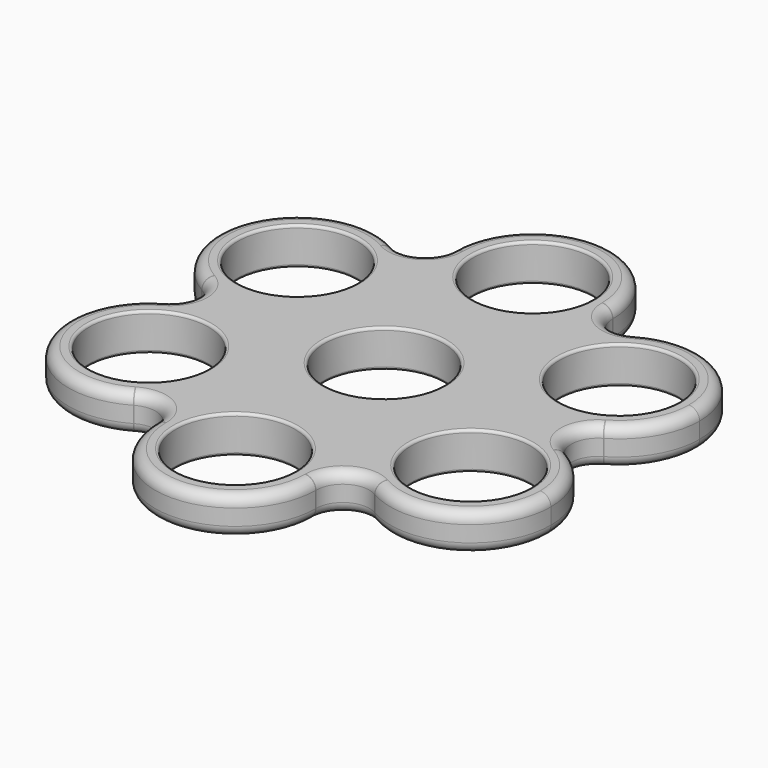
from build123d import *

# Parameters (mm, degrees)
F0_R     = 11.175
F1_DEPTH = 7
F2_R     = 5
F3_R     = 0.5
F4_R     = 2


# Not quite as in the source:
# - a feature names something its author has since deleted; it is built from what else it names


with BuildPart() as f1:
    # F0 (on Top) → F1 (new body)
    with BuildSketch(Plane.XY):
        with BuildLine():
            Line((15, 0), (15, 8.6602540378))
            Line((15, 8.6602540378), (7.5, 12.9903810568))
            Line((7.5, 12.9903810568), (0, 17.3205080757))
            Line((0, 17.3205080757), (-7.5, 12.9903810568))
            Line((-7.5, 12.9903810568), (-15, 8.6602540378))
            Line((-15, 8.6602540378), (-15, 0))
            Line((-15, 0), (-11.175, 0))
            ThreePointArc((-11.175, 0), (0, 11.175), (11.175, 0))
            Line((11.175, 0), (15, 0))
        make_face()
        with BuildLine():
            Line((15, 25.9807621135), (15, 34.7227789462))
            ThreePointArc((15, 34.7227789462), (0, 19.7227789462), (-15, 34.7227789462))
            Line((-15, 34.7227789462), (-15, 25.9807621135))
            Line((-15, 25.9807621135), (0, 17.3205080757))
            Line((0, 17.3205080757), (15, 25.9807621135))
        make_face()
        with BuildLine():
            ThreePointArc((-15, 34.7227789462), (0, 19.7227789462), (15, 34.7227789462))
            ThreePointArc((15, 34.7227789462), (0, 49.7227789462), (-15, 34.7227789462))
        make_face()
        with Locations((0, 34.7227789462)):
            Circle(F0_R, mode=Mode.SUBTRACT)
        with BuildLine():
            ThreePointArc((-15.0708086574, 17.3613894731), (-17.0804276006, 24.8613894731), (-22.5708086574, 30.3517705298))
            ThreePointArc((-22.5708086574, 30.3517705298), (-43.0611897141, 24.8613894731), (-37.5708086574, 4.3710084163))
            ThreePointArc((-37.5708086574, 4.3710084163), (-22.5708086574, 4.3710084163), (-15.0708086574, 17.3613894731))
        make_face()
        with Locations((-30.0708086574, 17.3613894731)):
            Circle(F0_R, mode=Mode.SUBTRACT)
        with BuildLine():
            ThreePointArc((-15, -34.7227789462), (0, -49.7227789462), (15, -34.7227789462))
            ThreePointArc((15, -34.7227789462), (0, -19.7227789462), (-15, -34.7227789462))
        make_face()
        with Locations((0, -34.7227789462)):
            Circle(F0_R, mode=Mode.SUBTRACT)
        with BuildLine():
            Line((15, -34.7227789462), (15, -25.9807621135))
            Line((15, -25.9807621135), (0, -17.3205080757))
            Line((0, -17.3205080757), (-15, -25.9807621135))
            Line((-15, -25.9807621135), (-15, -34.7227789462))
            ThreePointArc((-15, -34.7227789462), (0, -19.7227789462), (15, -34.7227789462))
        make_face()
        Polygon((30, 0), (15, 8.6602540378), (15, 0), (15, -8.6602540378), align=None)
        with BuildLine():
            ThreePointArc((-15.0708086574, -17.3613894731), (-22.5708086574, -4.3710084163), (-37.5708086574, -4.3710084163))
            ThreePointArc((-37.5708086574, -4.3710084163), (-43.0611897141, -24.8613894731), (-22.5708086574, -30.3517705298))
            ThreePointArc((-22.5708086574, -30.3517705298), (-17.0804276006, -24.8613894731), (-15.0708086574, -17.3613894731))
        make_face()
        with Locations((-30.0708086574, -17.3613894731)):
            Circle(F0_R, mode=Mode.SUBTRACT)
        with BuildLine():
            Line((-15, -8.6602540378), (-30, 0))
            Line((-30, 0), (-37.5708086574, -4.3710084163))
            ThreePointArc((-37.5708086574, -4.3710084163), (-22.5708086574, -4.3710084163), (-15.0708086574, -17.3613894731))
            ThreePointArc((-15.0708086574, -17.3613894731), (-17.0804276006, -24.8613894731), (-22.5708086574, -30.3517705298))
            Line((-22.5708086574, -30.3517705298), (-15, -25.9807621135))
            Line((-15, -25.9807621135), (-15, -8.6602540378))
        make_face()
        Polygon((-15, 0), (-15, 8.6602540378), (-30, 0), (-15, -8.6602540378), align=None)
        with BuildLine():
            Line((-15, 8.6602540378), (-15, 25.9807621135))
            Line((-15, 25.9807621135), (-22.5708086574, 30.3517705298))
            ThreePointArc((-22.5708086574, 30.3517705298), (-17.0804276006, 24.8613894731), (-15.0708086574, 17.3613894731))
            ThreePointArc((-15.0708086574, 17.3613894731), (-22.5708086574, 4.3710084163), (-37.5708086574, 4.3710084163))
            Line((-37.5708086574, 4.3710084163), (-30, 0))
            Line((-30, 0), (-15, 8.6602540378))
        make_face()
        Polygon((0, 17.3205080757), (-15, 25.9807621135), (-15, 8.6602540378), (-7.5, 12.9903810568), align=None)
        with BuildLine():
            Line((15, -8.6602540378), (15, 0))
            Line((15, 0), (11.175, 0))
            ThreePointArc((11.175, 0), (0, -11.175), (-11.175, 0))
            Line((-11.175, 0), (-15, 0))
            Line((-15, 0), (-15, -8.6602540378))
            Line((-15, -8.6602540378), (-7.5, -12.9903810568))
            Line((-7.5, -12.9903810568), (0, -17.3205080757))
            Line((0, -17.3205080757), (7.5, -12.9903810568))
            Line((7.5, -12.9903810568), (15, -8.6602540378))
        make_face()
        Polygon((15, 8.6602540378), (15, 25.9807621135), (0, 17.3205080757), (7.5, 12.9903810568), align=None)
        with BuildLine():
            Line((22.5708086574, 30.3517705298), (15, 25.9807621135))
            Line((15, 25.9807621135), (15, 8.6602540378))
            Line((15, 8.6602540378), (30, 0))
            Line((30, 0), (37.5708086574, 4.3710084163))
            ThreePointArc((37.5708086574, 4.3710084163), (17.0804276006, 9.8613894731), (22.5708086574, 30.3517705298))
        make_face()
        with BuildLine():
            ThreePointArc((45.0708086574, 17.3613894731), (37.5708086574, 30.3517705298), (22.5708086574, 30.3517705298))
            ThreePointArc((22.5708086574, 30.3517705298), (17.0804276006, 9.8613894731), (37.5708086574, 4.3710084163))
            ThreePointArc((37.5708086574, 4.3710084163), (43.0611897141, 9.8613894731), (45.0708086574, 17.3613894731))
        make_face()
        with Locations((30.0708086574, 17.3613894731)):
            Circle(F0_R, mode=Mode.SUBTRACT)
        with BuildLine():
            ThreePointArc((45.0708086574, -17.3613894731), (43.0611897141, -9.8613894731), (37.5708086574, -4.3710084163))
            ThreePointArc((37.5708086574, -4.3710084163), (17.0804276006, -9.8613894731), (22.5708086574, -30.3517705298))
            ThreePointArc((22.5708086574, -30.3517705298), (37.5708086574, -30.3517705298), (45.0708086574, -17.3613894731))
        make_face()
        with Locations((30.0708086574, -17.3613894731)):
            Circle(F0_R, mode=Mode.SUBTRACT)
        Polygon((15, -25.9807621135), (15, -8.6602540378), (7.5, -12.9903810568), (0, -17.3205080757), align=None)
        Polygon((-7.5, -12.9903810568), (-15, -8.6602540378), (-15, -25.9807621135), (0, -17.3205080757), align=None)
        with BuildLine():
            Line((37.5708086574, -4.3710084163), (30, 0))
            Line((30, 0), (15, -8.6602540378))
            Line((15, -8.6602540378), (15, -25.9807621135))
            Line((15, -25.9807621135), (22.5708086574, -30.3517705298))
            ThreePointArc((22.5708086574, -30.3517705298), (17.0804276006, -9.8613894731), (37.5708086574, -4.3710084163))
        make_face()
    extrude(amount=F1_DEPTH)

    # F2
    f2_edges = [f1.edges().sort_by_distance(p)[0] for p in [
        (-15, -25.980762, 3.5),
        (-30, 0, 3.5),
        (30, 0, 3.5),
        (15, -25.980762, 3.5),
        (15, 25.980762, 3.5),
        (-15, 25.980762, 3.5),
    ]]
    fillet(f2_edges, radius=F2_R)

    # F3
    f3_edges = [f1.edges().sort_by_distance(p)[0] for p in [
        (-11.175, 34.722779, 7),
        (-11.175, 0, 7),
        (-11.175, 34.722779, 0),
        (-11.175, 0, 0),
        (-41.245809, -17.361389, 7),
        (-41.245809, 17.361389, 0),
        (-11.175, -34.722779, 0),
        (-41.245809, -17.361389, 0),
        (-11.175, -34.722779, 7),
        (-41.245809, 17.361389, 7),
        (18.895809, 17.361389, 7),
        (18.895809, -17.361389, 7),
        (18.895809, 17.361389, 0),
        (18.895809, -17.361389, 0),
    ]]
    fillet(f3_edges, radius=F3_R)

    # F4
    f4_edges = [f1.edges().sort_by_distance(p)[0] for p in [
        (-17.5, 30.310889, 0),
        (-15, 34.641016, 3.5),
        (-22.5, 30.310889, 3.5),
        (-17.5, 30.310889, 7),
        (-15, 34.681898, 0),
        (-15, 34.722779, 3.5),
        (-15, 34.681898, 7),
        (15, 34.722779, 3.5),
        (0, 49.722779, 0),
        (0, 49.722779, 7),
        (15, 34.681898, 0),
        (15, 34.641016, 3.5),
        (15, 34.681898, 7),
        (17.5, 30.310889, 0),
        (22.5, 30.310889, 3.5),
        (17.5, 30.310889, 7),
        (-43.06119, -24.861389, 7),
        (-43.06119, -24.861389, 0),
        (-22.535404, -30.33133, 0),
        (-17.5, -30.310889, 0),
        (-15, -34.681898, 0),
        (-37.535404, -4.350568, 0),
        (0, -49.722779, 0),
        (-35, 0, 0),
        (15, -34.681898, 0),
        (-37.535404, 4.350568, 0),
        (17.5, -30.310889, 0),
        (-43.06119, 24.861389, 0),
        (22.535404, -30.33133, 0),
        (-22.535404, 30.33133, 0),
        (43.06119, -24.861389, 0),
        (37.535404, -4.350568, 0),
        (35, 0, 0),
        (37.535404, 4.350568, 0),
        (43.06119, 24.861389, 0),
        (22.535404, 30.33133, 0),
        (-22.535404, -30.33133, 7),
        (-17.5, -30.310889, 7),
        (-15, -34.681898, 7),
        (-37.535404, -4.350568, 7),
        (0, -49.722779, 7),
        (-35, 0, 7),
        (15, -34.681898, 7),
        (-37.535404, 4.350568, 7),
        (17.5, -30.310889, 7),
        (-43.06119, 24.861389, 7),
        (22.535404, -30.33133, 7),
        (-22.535404, 30.33133, 7),
        (43.06119, -24.861389, 7),
        (37.535404, -4.350568, 7),
        (35, 0, 7),
        (37.535404, 4.350568, 7),
        (43.06119, 24.861389, 7),
        (22.535404, 30.33133, 7),
    ]]
    fillet(f4_edges, radius=F4_R)


solid = f1.part
